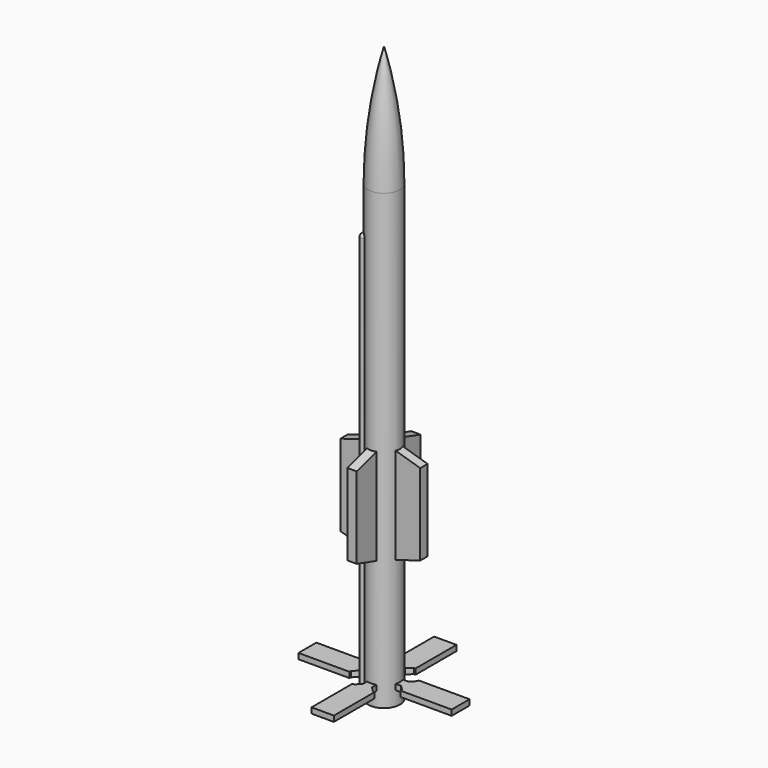
from build123d import *

# Parameters (mm, degrees)
F4_DEPTH     = 0.2
F6_DEPTH     = 0.2430555556
F7_COUNT     = 4
F10_DEPTH    = 17.3611111111
F11_T4_ANGLE = 107.9477893391
F11_S5_R     = 0.1388888889
F11_T6_DEPTH = 2
F12_R        = 0.138789
F13_SIZE     = 0.2083333333


# Not quite as in the source:
# - a fillet or chamfer that OpenCascade refuses, or shapes differently, is made with other operations: its cross-section is extruded or revolved along the edge and cut away or added
# - a fillet or chamfer is up to 0.001 mm smaller than in the source, because OpenCascade refuses the exact size
# - a feature names something its author has since deleted; it is built from what else it names


with BuildPart() as f2:
    # F1 (on Front) → F2 (revolve)
    with BuildSketch(Plane.XZ):
        with BuildLine():
            Line((0, 25), (0, 0))
            Line((0, 0), (0.6944444444, 0))
            Line((0.6944444444, 0), (0.6944444444, 19.7222222222))
            ThreePointArc((0.6944444444, 19.7222222222), (0.5200883354, 22.3838566523), (0, 25))
        make_face()
    revolve(axis=Axis((0, 0, 12.5), (0, 0, 1)))

    # F3 (on Front) → F4 (join, symmetric)
    with BuildSketch(Plane.XZ):
        Polygon((0, 10), (0, 0.625), (3.3333333333, 0.625), (3.3333333333, 0.8680555556), (0.4, 0.8680555556), (0.4, 5.5366666667), (1.7361111111, 5.9375), (1.7361111111, 9.4791666667), align=None)
    extrude(amount=F4_DEPTH, both=True)

    # F5 (on face) → F6 (join, through all)
    with BuildSketch(Plane(origin=(0, 0, 0.625), x_dir=(1, 0, 0), z_dir=(0, 0, -1))):
        Polygon((1.1111111111, -0.4861111111), (3.3333333333, -0.4861111111), (3.3333333333, 0.4861111111), (1.1111111111, 0.4861111111), (1.1111111111, 0), align=None)
    extrude(amount=-F6_DEPTH)

    # F7: F2 ×4 about axis
    f7_axis = Axis((0, 0, 0), (0, 0, 1))


with BuildPart() as f2_1:
    add(f2.part)
    for i in range(1, F7_COUNT):
        add(f2.part.rotate(f7_axis, i * 360 / F7_COUNT))

    # F9 (on offset) → F10 (join)
    with BuildSketch(Plane.XY.offset(0.5208333333)):
        with BuildLine():
            Line((-0.3928371007, -0.589255651), (-0.0580600084, -0.2544785587))
            Line((-0.0580600084, -0.2544785587), (-0.2544785587, -0.0580600084))
            Line((-0.2544785587, -0.0580600084), (-0.589255651, -0.3928371007))
            ThreePointArc((-0.589255651, -0.3928371007), (-0.589255651, -0.589255651), (-0.3928371007, -0.589255651))
        make_face()
    extrude(amount=F10_DEPTH)

    # F11: chamfer of 0.2 on 1 edges, made by hand


with BuildPart() as f11_tool2:
    # F11_s3 → F11_t4 (revolve)
    with BuildSketch(Plane(origin=(0, 0, 0), x_dir=(0, 0, 1), z_dir=(0.1559844343, 0.9877595134, 0))):
        with BuildLine():
            Line((0.3151764791, -0.6887875902), (0.5264901876, -0.9001012987))
            Line((0.5264901876, -0.9001012987), (0.5304901876, -0.9001012987))
            ThreePointArc((0.5304901876, -0.9001012987), (0.5248333333, -0.7972728716), (0.5248333333, -0.6944444444))
            Line((0.5248333333, -0.6944444444), (0.5208333333, -0.6904444444))
            ThreePointArc((0.5208333333, -0.6904444444), (0.4180049062, -0.6904444444), (0.3151764791, -0.6847875902))
            Line((0.3151764791, -0.6847875902), (0.3151764791, -0.6887875902))
        make_face()
    revolve(axis=Axis((0, 0, 0.5208333333), (0, 0, 1)), revolution_arc=F11_T4_ANGLE)

    # F11_s5 → F11_t6 (intersect, symmetric)
    with BuildSketch(Plane.XY.offset(0.4)):
        with Locations((-0.4910463758, -0.4910463758)):
            Circle(F11_S5_R)
    extrude(amount=F11_T6_DEPTH, both=True, mode=Mode.INTERSECT)


with BuildPart() as f2_2:
    add(f2_1.part)

    # F11_t1: union F11_tool2
    add(f11_tool2.part)

    # F12 (radius 0.1388888889 in the source; OpenCascade refuses exactly that, so slightly less here)
    f12_edges = [f2_2.edges().sort_by_distance(p)[0] for p in [
        (-0.589256, -0.589256, 17.881944),
    ]]
    fillet(f12_edges, radius=F12_R)

    # F13
    f13_edges = [f2_2.edges().sort_by_distance(p)[0] for p in [
        (1.111111, -0.2, 0.746528),
        (1.111111, 0.2, 0.746528),
        (-0.2, -1.111111, 0.746528),
        (0.2, -1.111111, 0.746528),
        (-1.111111, 0.2, 0.746528),
        (-0.2, 1.111111, 0.746528),
        (0.2, 1.111111, 0.746528),
        (-1.111111, -0.2, 0.746528),
    ]]
    chamfer(f13_edges, length=F13_SIZE)


solid = f2_2.part
